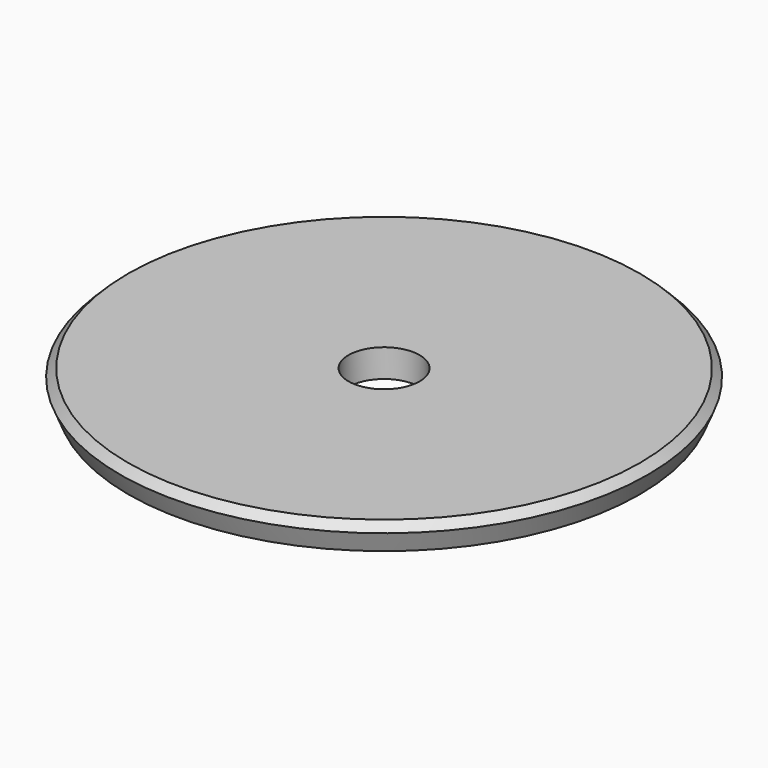
from build123d import *

# Parameters (mm, degrees)
F0_R     = 50.8
F1_DEPTH = 5
F2_R     = 6.35
F3_DEPTH = 5.001
F5_SIZE  = 5.08


# Not quite as in the source:
# - a fillet or chamfer that OpenCascade refuses, or shapes differently, is made with other operations: its cross-section is extruded or revolved along the edge and cut away or added


with BuildPart() as f1:
    # F0 (on Top) → F1 (new body)
    with BuildSketch(Plane.XY):
        Circle(F0_R)
    extrude(amount=F1_DEPTH)

    # F2 (on face) → F3 (cut, through all)
    with BuildSketch(Plane.XY.offset(5)):
        Circle(F2_R)
    extrude(amount=-F3_DEPTH, mode=Mode.SUBTRACT)

    # F4: chamfer of 5.08 on 1 edges, made by hand

    # F4_s1 → F4_t2 (revolve, cut)
    with BuildSketch(Plane.XZ):
        Polygon((50.8, -0.08), (45.72, 5), (50.8, 5), align=None)
    revolve(axis=Axis((0, 0, 5), (0, 0, 1)), mode=Mode.SUBTRACT)

    # F5
    f5_edges = [f1.edges().sort_by_distance(p)[0] for p in [
        (-50.72, 0, 0),
    ]]
    chamfer(f5_edges, length=F5_SIZE)


solid = f1.part
